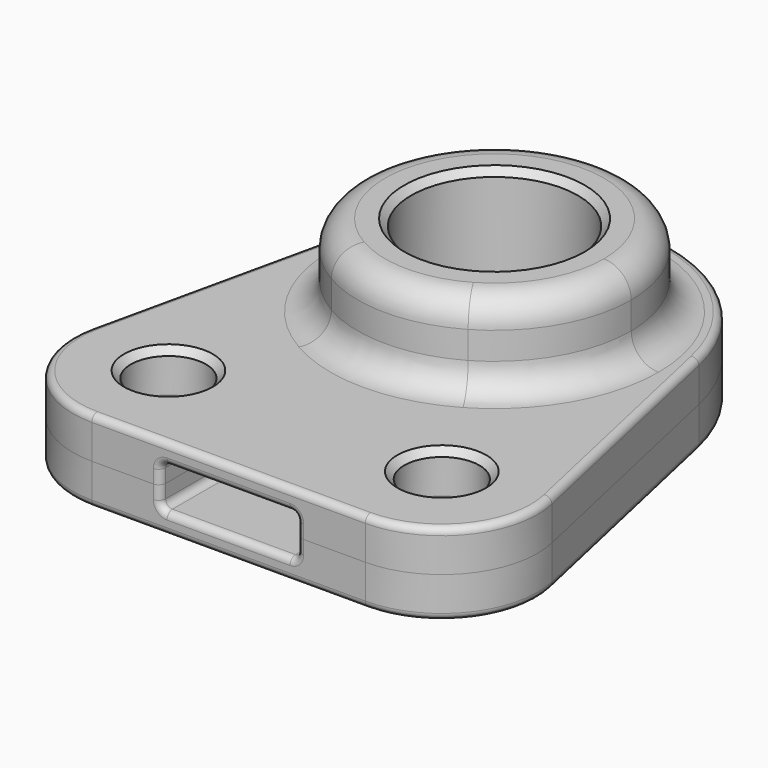
from build123d import *

# Parameters (mm, degrees)
F0_R      = 2.75
F0_R_2    = 9.25
F1_DEPTH  = 3
F0_R_3    = 6.1
F2_DEPTH  = 9
F3_DEPTH  = 1.5
F4_R      = 2
F5_SIZE   = 0.5
F0_R_4    = 5
F6_DEPTH  = 3
F7_DEPTH  = 1.5
F8_F1_R   = 0.5
F8_F2_R   = 0.5
F8_F3_R   = 0.5
F8_2_F1_R = 0.5
F8_2_F2_R = 0.5
F8_2_F3_R = 0.5


with BuildPart() as f1:
    # F0 (on Top) → F1 (new body)
    with BuildSketch(Plane.XY):
        with BuildLine():
            ThreePointArc((-15, 8.6602540378), (-15, 25.9807621135), (0, 17.3205080757))
            ThreePointArc((0, 17.3205080757), (-1.3397459622, 12.3205080757), (-5, 8.6602540378))
            Line((-5, 8.6602540378), (-5, -7))
            Line((-5, -7), (0, -7))
            ThreePointArc((0, -7), (5.4608120733, -4.3794441999), (6.8329490747, 1.520133857))
            Line((6.8329490747, 1.520133857), (2.6897625672, 20.1436138101))
            ThreePointArc((2.6897625672, 20.1436138101), (-10, 30.3205080757), (-22.6897625672, 20.1436138101))
            Line((-22.6897625672, 20.1436138101), (-26.8329490747, 1.520133857))
            ThreePointArc((-26.8329490747, 1.520133857), (-25.4608120733, -4.3794441999), (-20, -7))
            Line((-20, -7), (-15, -7))
            Line((-15, -7), (-15, 8.6602540378))
        make_face()
        with Locations((-20, 0)):
            Circle(F0_R, mode=Mode.SUBTRACT)
        Circle(F0_R, mode=Mode.SUBTRACT)
        with BuildLine():
            ThreePointArc((-5, 8.6602540378), (-1.3397459622, 12.3205080757), (0, 17.3205080757))
            ThreePointArc((0, 17.3205080757), (-15, 25.9807621135), (-15, 8.6602540378))
            ThreePointArc((-15, 8.6602540378), (-10, 7.3205080757), (-5, 8.6602540378))
        make_face()
        with Locations((-10, 17.3205080757)):
            Circle(F0_R_2, mode=Mode.SUBTRACT)
        with BuildLine():
            ThreePointArc((-5, 8.6602540378), (-10, 7.3205080757), (-15, 8.6602540378))
            Line((-15, 8.6602540378), (-15, -7))
            Line((-15, -7), (-5, -7))
            Line((-5, -7), (-5, 8.6602540378))
        make_face()
    extrude(amount=F1_DEPTH)

    # F0 (on Top) → F2 (join)
    with BuildSketch(Plane.XY):
        with BuildLine():
            ThreePointArc((-5, 8.6602540378), (-1.3397459622, 12.3205080757), (0, 17.3205080757))
            ThreePointArc((0, 17.3205080757), (-15, 25.9807621135), (-15, 8.6602540378))
            ThreePointArc((-15, 8.6602540378), (-10, 7.3205080757), (-5, 8.6602540378))
        make_face()
        with Locations((-10, 17.3205080757)):
            Circle(F0_R_2, mode=Mode.SUBTRACT)
        with Locations((-10, 17.3205080757)):
            Circle(F0_R_2)
        with Locations((-10, 17.3205080757)):
            Circle(F0_R_3, mode=Mode.SUBTRACT)
    extrude(amount=F2_DEPTH)

    # F0 (on Top) → F3 (cut)
    with BuildSketch(Plane.XY):
        with BuildLine():
            ThreePointArc((-5, 8.6602540378), (-1.3397459622, 12.3205080757), (0, 17.3205080757))
            ThreePointArc((0, 17.3205080757), (-15, 25.9807621135), (-15, 8.6602540378))
            ThreePointArc((-15, 8.6602540378), (-10, 7.3205080757), (-5, 8.6602540378))
        make_face()
        with Locations((-10, 17.3205080757)):
            Circle(F0_R_2, mode=Mode.SUBTRACT)
        with Locations((-10, 17.3205080757)):
            Circle(F0_R_2)
        with Locations((-10, 17.3205080757)):
            Circle(F0_R_3, mode=Mode.SUBTRACT)
        with BuildLine():
            ThreePointArc((-5, 8.6602540378), (-10, 7.3205080757), (-15, 8.6602540378))
            Line((-15, 8.6602540378), (-15, -7))
            Line((-15, -7), (-5, -7))
            Line((-5, -7), (-5, 8.6602540378))
        make_face()
    extrude(amount=F3_DEPTH, mode=Mode.SUBTRACT)

    # F4
    f4_edges = [f1.edges().sort_by_distance(p)[0] for p in [
        (-20, 17.320508, 3),
        (-20, 17.320508, 9),
    ]]
    fillet(f4_edges, radius=F4_R)

    # F5
    f5_edges = [f1.edges().sort_by_distance(p)[0] for p in [
        (-16.1, 17.320508, 9),
        (-22.75, 0, 3),
        (-2.75, 0, 3),
    ]]
    chamfer(f5_edges, length=F5_SIZE)

    # F8: fillet of radius 0.5 on 10 edges, made by hand

    # F8_f1
    f8_f1_edges = [f1.edges().sort_by_distance(p)[0] for p in [
        (-5, 0.8301270189, 1.5),
        (-15, 0.8301270189, 1.5),
    ]]
    fillet(f8_f1_edges, radius=F8_F1_R)

    # F8_f2
    f8_f2_edges = [f1.edges().sort_by_distance(p)[0] for p in [
        (-25.4608120733, -4.3794441999, 3),
        (-24.7613558209, 10.8318738336, 3),
        (-10, 30.3205080757, 3),
        (4.7613558209, 10.8318738336, 3),
        (-10, -7, 3),
        (5.4608120733, -4.3794441999, 3),
    ]]
    fillet(f8_f2_edges, radius=F8_F2_R)

    # F8_f3
    f8_f3_edges = [f1.edges().sort_by_distance(p)[0] for p in [
        (-15, -7, 0.5),
        (-10, -7, 1.5),
        (-14.8535533906, -7, 1.3535533906),
        (-5.1464466094, -7, 1.3535533906),
    ]]
    fillet(f8_f3_edges, radius=F8_F3_R)


with BuildPart() as f6:
    # F0 (on Top) → F6 (new body)
    with BuildSketch(Plane.XY):
        with BuildLine():
            ThreePointArc((-15, 8.6602540378), (-15, 25.9807621135), (0, 17.3205080757))
            ThreePointArc((0, 17.3205080757), (-1.3397459622, 12.3205080757), (-5, 8.6602540378))
            Line((-5, 8.6602540378), (-5, -7))
            Line((-5, -7), (0, -7))
            ThreePointArc((0, -7), (5.4608120733, -4.3794441999), (6.8329490747, 1.520133857))
            Line((6.8329490747, 1.520133857), (2.6897625672, 20.1436138101))
            ThreePointArc((2.6897625672, 20.1436138101), (-10, 30.3205080757), (-22.6897625672, 20.1436138101))
            Line((-22.6897625672, 20.1436138101), (-26.8329490747, 1.520133857))
            ThreePointArc((-26.8329490747, 1.520133857), (-25.4608120733, -4.3794441999), (-20, -7))
            Line((-20, -7), (-15, -7))
            Line((-15, -7), (-15, 8.6602540378))
        make_face()
        with Locations((-20, 0)):
            Circle(F0_R, mode=Mode.SUBTRACT)
        Circle(F0_R, mode=Mode.SUBTRACT)
        with BuildLine():
            ThreePointArc((-5, 8.6602540378), (-1.3397459622, 12.3205080757), (0, 17.3205080757))
            ThreePointArc((0, 17.3205080757), (-15, 25.9807621135), (-15, 8.6602540378))
            ThreePointArc((-15, 8.6602540378), (-10, 7.3205080757), (-5, 8.6602540378))
        make_face()
        with Locations((-10, 17.3205080757)):
            Circle(F0_R_2, mode=Mode.SUBTRACT)
        with Locations((-10, 17.3205080757)):
            Circle(F0_R_2)
        with Locations((-10, 17.3205080757)):
            Circle(F0_R_3, mode=Mode.SUBTRACT)
        with BuildLine():
            ThreePointArc((-5, 8.6602540378), (-10, 7.3205080757), (-15, 8.6602540378))
            Line((-15, 8.6602540378), (-15, -7))
            Line((-15, -7), (-5, -7))
            Line((-5, -7), (-5, 8.6602540378))
        make_face()
        with Locations((-10, 17.3205080757)):
            Circle(F0_R_3)
        with Locations((-10, 17.3205080757)):
            Circle(F0_R_4, mode=Mode.SUBTRACT)
        with Locations((-10, 17.3205080757)):
            Circle(F0_R_4)
    extrude(amount=-F6_DEPTH)

    # F0 (on Top) → F7 (cut)
    with BuildSketch(Plane.XY):
        with BuildLine():
            ThreePointArc((-5, 8.6602540378), (-10, 7.3205080757), (-15, 8.6602540378))
            Line((-15, 8.6602540378), (-15, -7))
            Line((-15, -7), (-5, -7))
            Line((-5, -7), (-5, 8.6602540378))
        make_face()
        with BuildLine():
            ThreePointArc((-5, 8.6602540378), (-1.3397459622, 12.3205080757), (0, 17.3205080757))
            ThreePointArc((0, 17.3205080757), (-15, 25.9807621135), (-15, 8.6602540378))
            ThreePointArc((-15, 8.6602540378), (-10, 7.3205080757), (-5, 8.6602540378))
        make_face()
        with Locations((-10, 17.3205080757)):
            Circle(F0_R_2, mode=Mode.SUBTRACT)
    extrude(amount=-F7_DEPTH, mode=Mode.SUBTRACT)

    # F8#2: fillet of radius 0.5 on 12 edges, made by hand

    # F8_2_f1
    f8_2_f1_edges = [f6.edges().sort_by_distance(p)[0] for p in [
        (-15, 0.8301270189, -1.5),
        (-5, 0.8301270189, -1.5),
    ]]
    fillet(f8_2_f1_edges, radius=F8_2_F1_R)

    # F8_2_f2
    f8_2_f2_edges = [f6.edges().sort_by_distance(p)[0] for p in [
        (-24.7613558209, 10.8318738336, -3),
        (-25.4608120733, -4.3794441999, -3),
        (-10, -7, -3),
        (5.4608120733, -4.3794441999, -3),
        (4.7613558209, 10.8318738336, -3),
        (-10, 30.3205080757, -3),
        (-22.75, 0, -3),
        (-2.75, 0, -3),
    ]]
    fillet(f8_2_f2_edges, radius=F8_2_F2_R)

    # F8_2_f3
    f8_2_f3_edges = [f6.edges().sort_by_distance(p)[0] for p in [
        (-15, -7, -0.5),
        (-10, -7, -1.5),
        (-14.8535533906, -7, -1.3535533906),
        (-5.1464466094, -7, -1.3535533906),
    ]]
    fillet(f8_2_f3_edges, radius=F8_2_F3_R)


solid = Compound([f1.part, f6.part])
